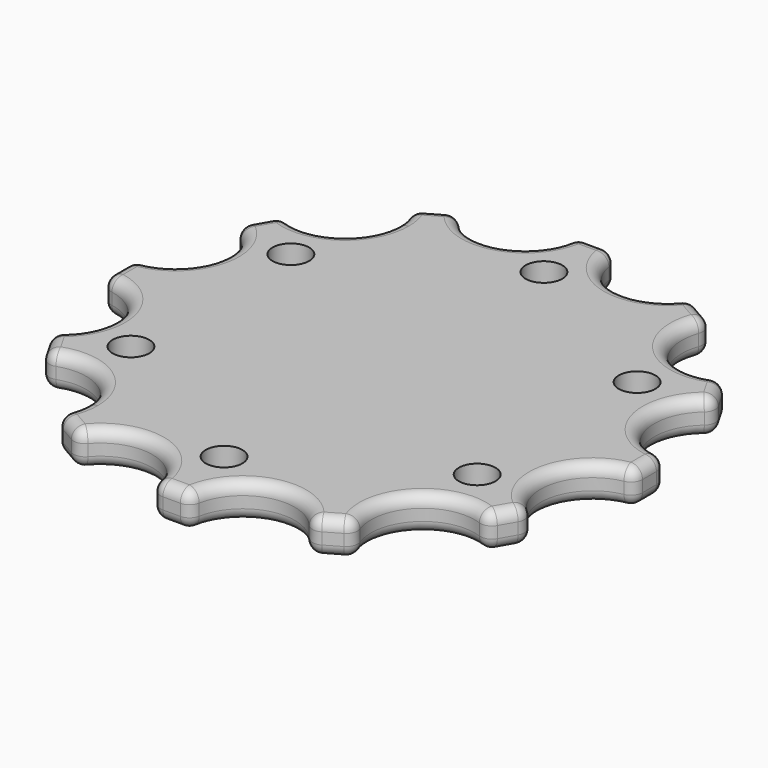
from build123d import *

# Parameters (mm, degrees)
F1_R     = 3.175
F2_DEPTH = 6
F0_R     = 3.175
F3_DEPTH = 1.5
F4_F1_R  = 2
F4_F2_R  = 2
F4_F3_R  = 2
F4_F4_R  = 2
F4_F5_R  = 2
F4_F6_R  = 2
F4_F7_R  = 2
F4_F8_R  = 2
F4_F9_R  = 2
F4_F10_R = 2
F4_F11_R = 2
F4_F12_R = 2
F4_F13_R = 2
F4_F14_R = 2
F4_F15_R = 2
F4_F16_R = 2
F4_F17_R = 2
F4_F18_R = 2
F4_F19_R = 2
F4_F20_R = 2
F4_F21_R = 2
F4_F22_R = 2
F4_F23_R = 2
F4_F24_R = 2
F4_F25_R = 2
F4_F26_R = 2


# Not quite as in the source:
# - a feature of the source that left no trace in its solid (it failed there, or was rolled back) is left out


with BuildPart() as f2:
    # F1 (on face) → F2 (new body)
    with BuildSketch(Plane.XY):
        with BuildLine():
            Line((46, -3.3256628518), (46, 3.3256628518))
            ThreePointArc((46, 3.3256628518), (37.3066675634, 9.9962914459), (41.5, 20.1198914859))
            Line((41.5, 20.1198914859), (38.1743371482, 25.8801085141))
            ThreePointArc((38.1743371482, 25.8801085141), (27.3103761175, 27.3103761175), (25.8801085141, 38.1743371482))
            Line((25.8801085141, 38.1743371482), (20.1198914859, 41.5))
            ThreePointArc((20.1198914859, 41.5), (9.9962914459, 37.3066675634), (3.3256628518, 46))
            Line((3.3256628518, 46), (-3.3256628518, 46))
            ThreePointArc((-3.3256628518, 46), (-9.9962914459, 37.3066675634), (-20.1198914859, 41.5))
            Line((-20.1198914859, 41.5), (-25.8801085141, 38.1743371482))
            ThreePointArc((-25.8801085141, 38.1743371482), (-24.9810047116, 36.0037085541), (-24.6743371482, 33.6743371482))
            ThreePointArc((-24.6743371482, 33.6743371482), (-29.1743371482, 25.8801085141), (-38.1743371482, 25.8801085141))
            Line((-38.1743371482, 25.8801085141), (-41.5, 20.1198914859))
            ThreePointArc((-41.5, 20.1198914859), (-38.2057713659, 16.8256628518), (-37, 12.3256628518))
            ThreePointArc((-37, 12.3256628518), (-39.6360389693, 5.9617018212), (-46, 3.3256628518))
            Line((-46, 3.3256628518), (-46, -3.3256628518))
            ThreePointArc((-46, -3.3256628518), (-39.6360389693, -5.9617018212), (-37, -12.3256628518))
            ThreePointArc((-37, -12.3256628518), (-38.2057713659, -16.8256628518), (-41.5, -20.1198914859))
            Line((-41.5, -20.1198914859), (-38.1743371482, -25.8801085141))
            ThreePointArc((-38.1743371482, -25.8801085141), (-29.1743371482, -25.8801085141), (-24.6743371482, -33.6743371482))
            ThreePointArc((-24.6743371482, -33.6743371482), (-24.9810047116, -36.0037085541), (-25.8801085141, -38.1743371482))
            Line((-25.8801085141, -38.1743371482), (-20.1198914859, -41.5))
            ThreePointArc((-20.1198914859, -41.5), (-9.9962914459, -37.3066675634), (-3.3256628518, -46))
            Line((-3.3256628518, -46), (3.3256628518, -46))
            ThreePointArc((3.3256628518, -46), (9.9962914459, -37.3066675634), (20.1198914859, -41.5))
            Line((20.1198914859, -41.5), (25.8801085141, -38.1743371482))
            ThreePointArc((25.8801085141, -38.1743371482), (27.3103761175, -27.3103761175), (38.1743371482, -25.8801085141))
            Line((38.1743371482, -25.8801085141), (41.5, -20.1198914859))
            ThreePointArc((41.5, -20.1198914859), (37.3066675634, -9.9962914459), (46, -3.3256628518))
        make_face()
        with Locations((-30, -17.3205080757)):
            Circle(F1_R, mode=Mode.SUBTRACT)
        with Locations((0, -34.6410161514)):
            Circle(F1_R, mode=Mode.SUBTRACT)
        with Locations((30, -17.3205080757)):
            Circle(F1_R, mode=Mode.SUBTRACT)
        with Locations((-30, 17.3205080757)):
            Circle(F1_R, mode=Mode.SUBTRACT)
        with Locations((30, 17.3205080757)):
            Circle(F1_R, mode=Mode.SUBTRACT)
        with Locations((0, 34.6410161514)):
            Circle(F1_R, mode=Mode.SUBTRACT)
    extrude(amount=F2_DEPTH)

    # F0 (on Top) → F3 (join)
    with BuildSketch(Plane.XY):
        with Locations((-30, 17.3205080757)):
            Circle(F0_R)
        with Locations((0, 34.6410161514)):
            Circle(F0_R)
        with Locations((30, 17.3205080757)):
            Circle(F0_R)
        with Locations((30, -17.3205080757)):
            Circle(F0_R)
        with Locations((0, -34.6410161514)):
            Circle(F0_R)
        with Locations((-30, -17.3205080757)):
            Circle(F0_R)
    extrude(amount=F3_DEPTH)

    # F4: fillet of radius 2 on 60 edges, made by hand

    # F4_f1
    f4_f1_edges = [f2.edges().sort_by_distance(p)[0] for p in [
        (41.5, -20.1198914859, 3),
    ]]
    fillet(f4_f1_edges, radius=F4_F1_R)

    # F4_f2
    f4_f2_edges = [f2.edges().sort_by_distance(p)[0] for p in [
        (46, -3.3256628518, 3),
    ]]
    fillet(f4_f2_edges, radius=F4_F2_R)

    # F4_f3
    f4_f3_edges = [f2.edges().sort_by_distance(p)[0] for p in [
        (38.1743371482, -25.8801085141, 3),
    ]]
    fillet(f4_f3_edges, radius=F4_F3_R)

    # F4_f4
    f4_f4_edges = [f2.edges().sort_by_distance(p)[0] for p in [
        (46, 3.3256628518, 3),
    ]]
    fillet(f4_f4_edges, radius=F4_F4_R)

    # F4_f5
    f4_f5_edges = [f2.edges().sort_by_distance(p)[0] for p in [
        (25.8801085141, -38.1743371482, 3),
    ]]
    fillet(f4_f5_edges, radius=F4_F5_R)

    # F4_f6
    f4_f6_edges = [f2.edges().sort_by_distance(p)[0] for p in [
        (41.5, 20.1198914859, 3),
    ]]
    fillet(f4_f6_edges, radius=F4_F6_R)

    # F4_f7
    f4_f7_edges = [f2.edges().sort_by_distance(p)[0] for p in [
        (38.1743371482, 25.8801085141, 3),
    ]]
    fillet(f4_f7_edges, radius=F4_F7_R)

    # F4_f8
    f4_f8_edges = [f2.edges().sort_by_distance(p)[0] for p in [
        (25.8801085141, 38.1743371482, 3),
    ]]
    fillet(f4_f8_edges, radius=F4_F8_R)

    # F4_f9
    f4_f9_edges = [f2.edges().sort_by_distance(p)[0] for p in [
        (20.1198914859, 41.5, 3),
    ]]
    fillet(f4_f9_edges, radius=F4_F9_R)

    # F4_f10
    f4_f10_edges = [f2.edges().sort_by_distance(p)[0] for p in [
        (3.3256628518, 46, 3),
    ]]
    fillet(f4_f10_edges, radius=F4_F10_R)

    # F4_f11
    f4_f11_edges = [f2.edges().sort_by_distance(p)[0] for p in [
        (-3.3256628518, 46, 3),
    ]]
    fillet(f4_f11_edges, radius=F4_F11_R)

    # F4_f12
    f4_f12_edges = [f2.edges().sort_by_distance(p)[0] for p in [
        (-20.1198914859, 41.5, 3),
    ]]
    fillet(f4_f12_edges, radius=F4_F12_R)

    # F4_f13
    f4_f13_edges = [f2.edges().sort_by_distance(p)[0] for p in [
        (-25.8801085141, 38.1743371482, 3),
    ]]
    fillet(f4_f13_edges, radius=F4_F13_R)

    # F4_f14
    f4_f14_edges = [f2.edges().sort_by_distance(p)[0] for p in [
        (-38.1743371482, 25.8801085141, 3),
    ]]
    fillet(f4_f14_edges, radius=F4_F14_R)

    # F4_f15
    f4_f15_edges = [f2.edges().sort_by_distance(p)[0] for p in [
        (-41.5, 20.1198914859, 3),
    ]]
    fillet(f4_f15_edges, radius=F4_F15_R)

    # F4_f16
    f4_f16_edges = [f2.edges().sort_by_distance(p)[0] for p in [
        (-46, 3.3256628518, 3),
    ]]
    fillet(f4_f16_edges, radius=F4_F16_R)

    # F4_f17
    f4_f17_edges = [f2.edges().sort_by_distance(p)[0] for p in [
        (-46, -3.3256628518, 3),
    ]]
    fillet(f4_f17_edges, radius=F4_F17_R)

    # F4_f18
    f4_f18_edges = [f2.edges().sort_by_distance(p)[0] for p in [
        (-41.5, -20.1198914859, 3),
    ]]
    fillet(f4_f18_edges, radius=F4_F18_R)

    # F4_f19
    f4_f19_edges = [f2.edges().sort_by_distance(p)[0] for p in [
        (-38.1743371482, -25.8801085141, 3),
    ]]
    fillet(f4_f19_edges, radius=F4_F19_R)

    # F4_f20
    f4_f20_edges = [f2.edges().sort_by_distance(p)[0] for p in [
        (-25.8801085141, -38.1743371482, 3),
    ]]
    fillet(f4_f20_edges, radius=F4_F20_R)

    # F4_f21
    f4_f21_edges = [f2.edges().sort_by_distance(p)[0] for p in [
        (-20.1198914859, -41.5, 3),
    ]]
    fillet(f4_f21_edges, radius=F4_F21_R)

    # F4_f22
    f4_f22_edges = [f2.edges().sort_by_distance(p)[0] for p in [
        (-3.3256628518, -46, 3),
    ]]
    fillet(f4_f22_edges, radius=F4_F22_R)

    # F4_f23
    f4_f23_edges = [f2.edges().sort_by_distance(p)[0] for p in [
        (3.3256628518, -46, 3),
    ]]
    fillet(f4_f23_edges, radius=F4_F23_R)

    # F4_f24
    f4_f24_edges = [f2.edges().sort_by_distance(p)[0] for p in [
        (20.1198914859, -41.5, 3),
    ]]
    fillet(f4_f24_edges, radius=F4_F24_R)

    # F4_f25
    f4_f25_edges = [f2.edges().sort_by_distance(p)[0] for p in [
        (0, -46, 0),
    ]]
    fillet(f4_f25_edges, radius=F4_F25_R)

    # F4_f26
    f4_f26_edges = [f2.edges().sort_by_distance(p)[0] for p in [
        (0, -46, 6),
    ]]
    fillet(f4_f26_edges, radius=F4_F26_R)


solid = f2.part
